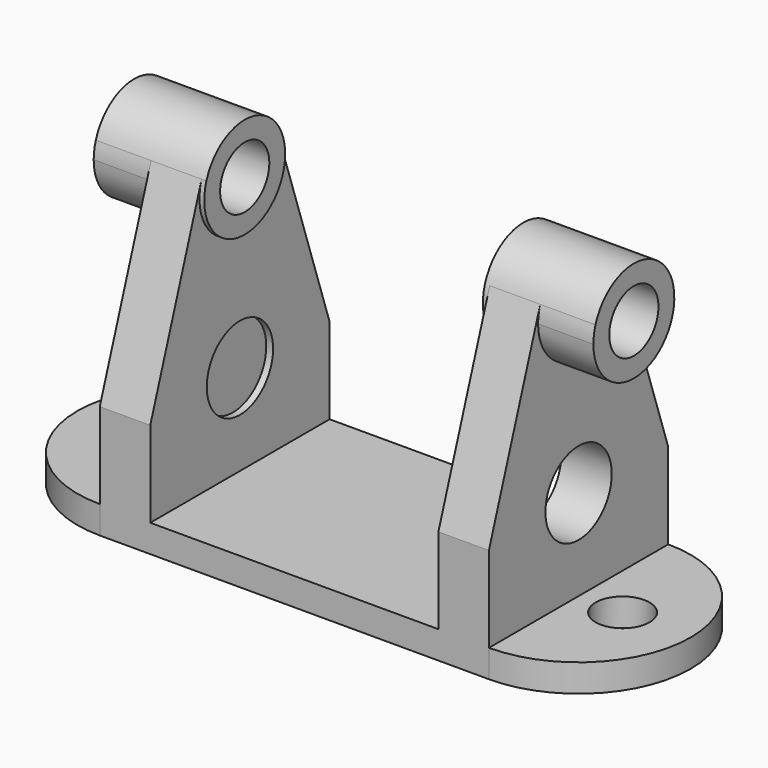
from build123d import *

# Parameters (mm, degrees)
F1_DEPTH  = 2
F3_DEPTH  = 14.08
F4_DEPTH  = 10.425
F6_DEPTH  = 4
F8_DEPTH  = 0.345
F9_R      = 2.225
F10_DEPTH = 8
F11_R     = 1.95
F12_DEPTH = 2
F14_DEPTH = 2
F16_R     = 3
F17_DEPTH = 25


with BuildPart() as f1:
    # F0 (on Top) → F1 (new body)
    with BuildSketch(Plane.XY):
        with BuildLine():
            Line((-14.08, -8.11), (0, -8.11))
            Line((0, -8.11), (0, 0))
            Line((0, 0), (0, 8.11))
            Line((0, 8.11), (-14.08, 8.11))
            ThreePointArc((-14.08, 8.11), (-22.19, 0), (-14.08, -8.11))
        make_face()
    extrude(amount=F1_DEPTH)

    # F2 (on Right) → F3 (join)
    with BuildSketch(Plane.YZ):
        with BuildLine():
            Line((-8.11, 8.21), (-8.11, 2))
            Line((-8.11, 2), (8.11, 2))
            Line((8.11, 2), (8.11, 8.21))
            Line((8.11, 8.21), (3.4687412656, 21.99766178))
            ThreePointArc((3.4687412656, 21.99766178), (0, 24.49), (-3.4687412656, 21.99766178))
            Line((-3.4687412656, 21.99766178), (-8.11, 8.21))
        make_face()
    extrude(amount=-F3_DEPTH)

    # F4 (cut): a face of the model
    f4_faces = [f1.faces().sort_by_distance(p)[0] for p in [
        (0, 0, 10.1553909867),
    ]]
    extrude(f4_faces, amount=-F4_DEPTH, mode=Mode.SUBTRACT)

    # F5 (on face) → F6 (join)
    with BuildSketch(Plane(origin=(-14.08, 0, 0), x_dir=(0, -1, 0), z_dir=(-1, 0, 0))):
        with BuildLine():
            ThreePointArc((-3.4687412656, 21.99766178), (-0.5916109228, 17.2181311602), (3.66, 20.83))
            ThreePointArc((3.66, 20.83), (3.6118688398, 21.4216109228), (3.4687412656, 21.99766178))
            ThreePointArc((3.4687412656, 21.99766178), (0, 24.49), (-3.4687412656, 21.99766178))
        make_face()
    extrude(amount=F6_DEPTH)

    # F7 (on face) → F8 (join)
    with BuildSketch(Plane.YZ.offset(-10.425)):
        with BuildLine():
            ThreePointArc((-3.4687412656, 21.99766178), (-0.5916109228, 17.2181311602), (3.66, 20.83))
            ThreePointArc((3.66, 20.83), (3.6118688398, 21.4216109228), (3.4687412656, 21.99766178))
            ThreePointArc((3.4687412656, 21.99766178), (0, 24.49), (-3.4687412656, 21.99766178))
        make_face()
    extrude(amount=F8_DEPTH)

    # F9 (on face) → F10 (cut)
    with BuildSketch(Plane(origin=(-18.08, 0, 0), x_dir=(0, -1, 0), z_dir=(-1, 0, 0))):
        with Locations((0, 20.83)):
            Circle(F9_R)
    extrude(amount=-F10_DEPTH, mode=Mode.SUBTRACT)

    # F11 (on face) → F12 (cut)
    with BuildSketch(Plane.XY.offset(2)):
        with Locations((-17.265, 0)):
            Circle(F11_R)
    extrude(amount=-F12_DEPTH, mode=Mode.SUBTRACT)

    # F13 (on face) → F14 (join)
    with BuildSketch(Plane.XY):
        Polygon((-10.425, 8.11), (-10.425, -8.11), (0, -8.11), (0, 0), (0, 8.11), align=None)
    extrude(amount=F14_DEPTH)

    # F15: F1 across plane


with BuildPart() as f1_1:
    add(f1.part)
    add(f1.part.mirror(Plane.YZ))

    # F16 (on face) → F17 (cut)
    with BuildSketch(Plane.YZ.offset(14.08)):
        with Locations((0, 8.5717271108)):
            Circle(F16_R)
    extrude(amount=-F17_DEPTH, mode=Mode.SUBTRACT)


solid = f1_1.part
